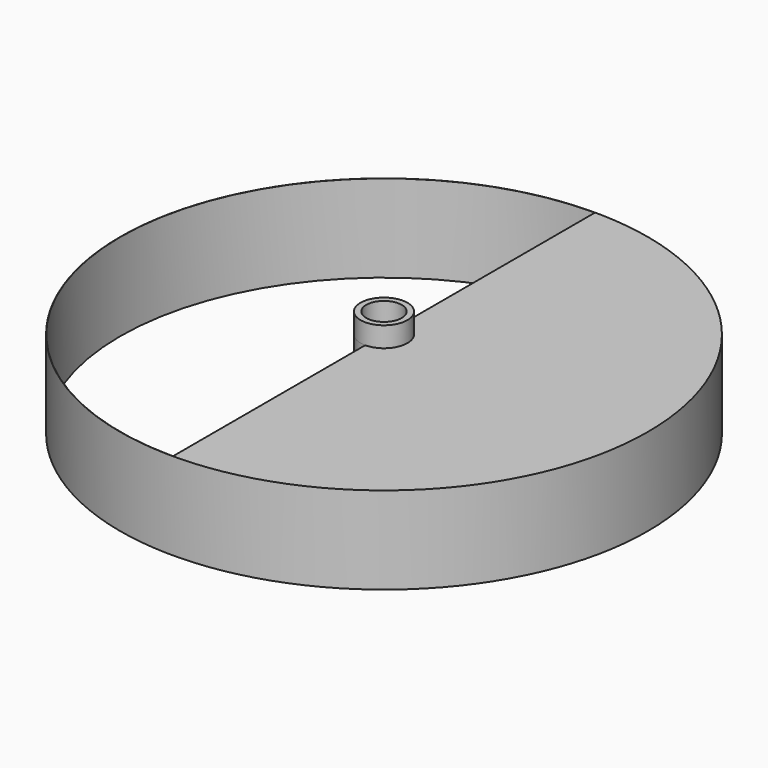
from build123d import *

# Parameters (mm, degrees)
F0_R          = 46.05
F1_DEPTH      = 15.24
F2_R          = 45.75
F3_DEPTH      = 12.7
F4_R          = 4.1
F5_DEPTH      = 3.53
F5_DEPTH_BACK = 1
F7_DEPTH      = 15.241
F8_R          = 3.1
F9_DEPTH      = 18.771


# Not quite as in the source:
# - after a boolean that leaves OpenCascade's solid faulty, fix() repairs it


with BuildPart() as f1:
    # F0 (on Top) → F1 (new body)
    with BuildSketch(Plane.XY):
        Circle(F0_R)
    extrude(amount=F1_DEPTH)

    # F2 (on Top) → F3 (cut)
    with BuildSketch(Plane.XY):
        Circle(F2_R)
    extrude(amount=F3_DEPTH, mode=Mode.SUBTRACT)

    # F4 (on face) → F5 (join, two sides)
    with BuildSketch(Plane.XY.offset(15.24)) as f5_sk:
        Circle(F4_R)
    extrude(amount=F5_DEPTH)
    extrude(f5_sk.sketch, amount=-F5_DEPTH_BACK)

    # F6 (on face) → F7 (cut, through all)
    with BuildSketch(Plane.XY.offset(15.24)):
        with BuildLine():
            Line((0, 4.1), (0, 46.03))
            ThreePointArc((0, 46.03), (-46.03, 0), (0, -46.03))
            Line((0, -46.03), (0, -4.1))
            ThreePointArc((0, -4.1), (-4.1, 0), (0, 4.1))
        make_face()
    extrude(amount=-F7_DEPTH, mode=Mode.SUBTRACT)

    add(f1.part.fix(), mode=Mode.REPLACE)

    # F8 (on face) → F9 (cut, through all)
    with BuildSketch(Plane.XY.offset(18.77)):
        Circle(F8_R)
    extrude(amount=-F9_DEPTH, mode=Mode.SUBTRACT)


solid = f1.part
